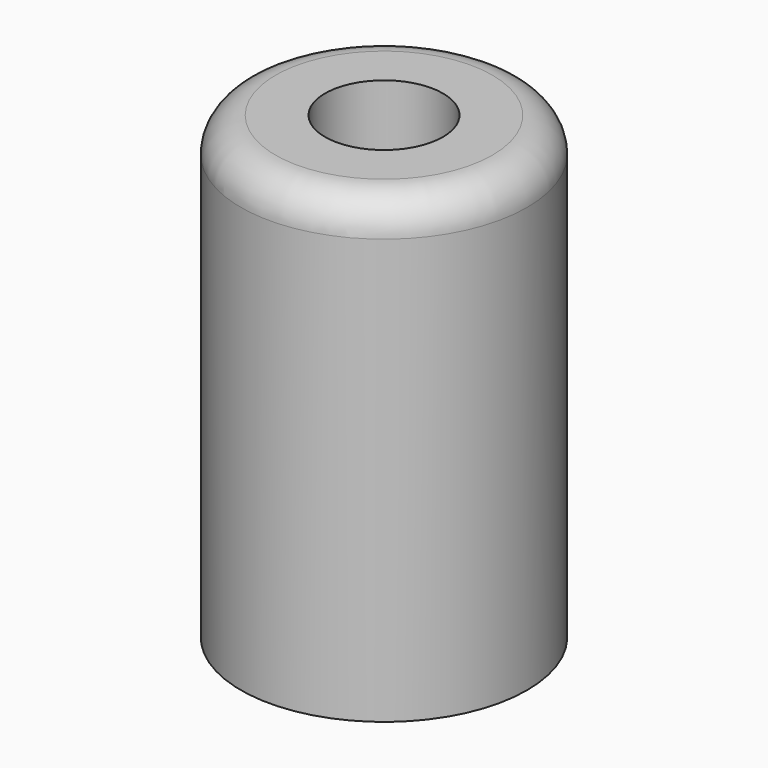
from build123d import *

# Parameters (mm, degrees)
F0_R         = 8.25
F1_DEPTH     = 26.5
F3_R         = 3.4
F4_DEPTH     = 19.7
F6_TEXT_SIZE = 6.3140144145
F7_DEPTH     = 3
F8_R         = 2


# Not quite as in the source:
# - Text() gives the source's letters only with a copy of the font that has no kerning and outlines rounded to 1/6400 em; it was checked with that copy


with BuildPart() as f1:
    # F0 (on Top) → F1 (new body)
    with BuildSketch(Plane.XY):
        Circle(F0_R)
    extrude(amount=F1_DEPTH)

    # F3 (on offset) → F4 (cut)
    with BuildSketch(Plane.XY.offset(26.5)):
        Circle(F3_R)
    extrude(amount=-F4_DEPTH, mode=Mode.SUBTRACT)

    # F6 (on offset) → F7 (cut)
    with BuildSketch(Plane(origin=(0, 0, 0), x_dir=(1, 0, 0), z_dir=(0, 0, -1))):
        with Locations((-5.8088940568, -1.3890831033)):
            Text('1/4', F6_TEXT_SIZE, font='Open Sans', font_style=FontStyle.BOLD, text_align=(TextAlign.LEFT, TextAlign.BOTTOM))
    extrude(amount=-F7_DEPTH, mode=Mode.SUBTRACT)

    # F8
    f8_edges = [f1.edges().sort_by_distance(p)[0] for p in [
        (-8.25, 0, 26.5),
    ]]
    fillet(f8_edges, radius=F8_R)


solid = f1.part
